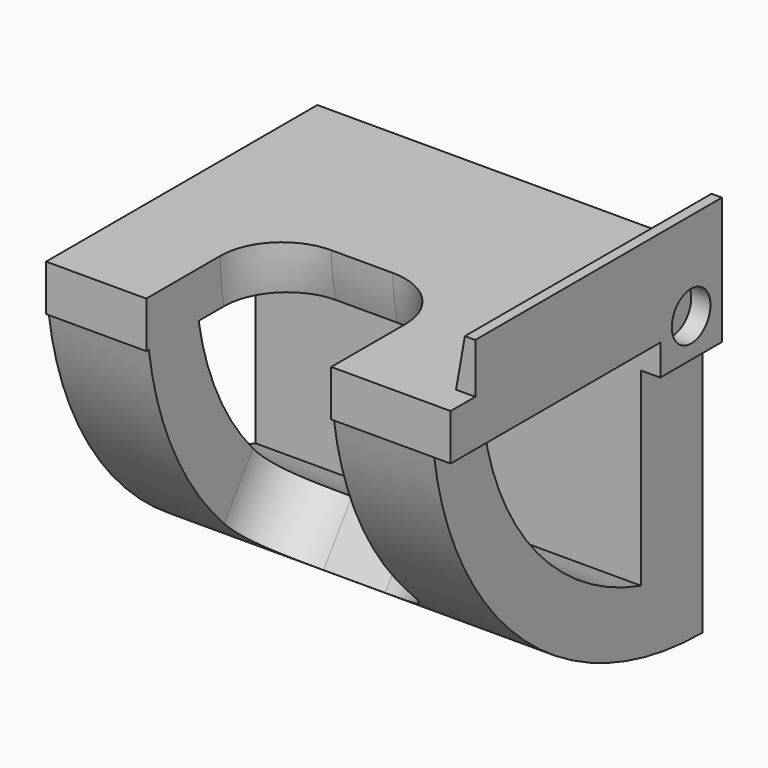
from build123d import *

# Parameters (mm, degrees)
F1_DEPTH      = 79.375
F4_DEPTH      = 19.05
F4_DEPTH_BACK = 19.05
F5_R          = 12.7
F7_W          = 9.525
F7_H          = 12.7
F8_DEPTH      = 3.175
F6_W          = 63.5
F6_H          = 10.3124
F6_R          = 4.9744809982
F9_DEPTH      = 3.9624
F10_SIZE2     = 1.818344
F10_SIZE      = 10.31239


# Not quite as in the source:
# - a fillet or chamfer is up to 0.001 mm smaller than in the source, because OpenCascade refuses the exact size


with BuildPart() as f1:
    # F0 (on Right) → F1 (new body)
    with BuildSketch(Plane.YZ):
        with BuildLine():
            Line((0, -9.525), (0, 0))
            Line((0, 0), (-57.15, 0))
            ThreePointArc((-57.15, 0), (-56.9498143774, -4.779240775), (-56.350659934, -9.525))
            Line((-56.350659934, -9.525), (-15.875, -9.525))
            Line((-15.875, -9.525), (0, -9.525))
        make_face()
        with BuildLine():
            ThreePointArc((-56.350659934, -9.525), (-56.9498143774, -4.779240775), (-57.15, 0))
            Line((-57.15, 0), (-69.85, 0))
            ThreePointArc((-69.85, 0), (-69.6866892703, -4.7736609169), (-69.1975207287, -9.525))
            Line((-69.1975207287, -9.525), (-56.350659934, -9.525))
        make_face()
        with BuildLine():
            Line((0, -57.15), (0, -9.525))
            Line((0, -9.525), (-15.875, -9.525))
            Line((-15.875, -9.525), (-15.875, -54.9008822789))
            ThreePointArc((-15.875, -54.9008822789), (-8.0167661111, -56.5849269781), (0, -57.15))
        make_face()
        with BuildLine():
            ThreePointArc((-69.1975207287, -9.525), (-69.6866892703, -4.7736609169), (-69.85, 0))
            Line((-69.85, 0), (-69.85, -9.525))
            Line((-69.85, -9.525), (-69.1975207287, -9.525))
        make_face()
        with BuildLine():
            ThreePointArc((-15.875, -54.9008822789), (-42.648319561, -38.042651572), (-56.350659934, -9.525))
            Line((-56.350659934, -9.525), (-69.1975207287, -9.525))
            ThreePointArc((-69.1975207287, -9.525), (-45.900442536, -52.6514185469), (0, -69.85))
            Line((0, -69.85), (0, -57.15))
            ThreePointArc((0, -57.15), (-8.0167661111, -56.5849269781), (-15.875, -54.9008822789))
        make_face()
    extrude(amount=-F1_DEPTH)

    # F3 (on offset) → F4 (cut, two sides)
    with BuildSketch(Plane.YZ.offset(-39.6875)) as f4_sk:
        with BuildLine():
            ThreePointArc((-21.853262225, -31.2096928874), (-33.7951127441, -17.5926221643), (-38.1, 0))
            Line((-38.1, 0), (-69.85, 0))
            Line((-69.85, 0), (-69.85, -9.525))
            Line((-69.85, -9.525), (-69.1975207287, -9.525))
            ThreePointArc((-69.1975207287, -9.525), (-59.6086170026, -36.4120210787), (-40.0643140791, -57.2177702936))
            Line((-40.0643140791, -57.2177702936), (-21.853262225, -31.2096928874))
        make_face()
        with BuildLine():
            ThreePointArc((-2.9503190018, -7.9502), (-3.1448391156, -6.5727258097), (-3.7131865837, -5.3029800181))
            Line((-3.7131865837, -5.3029800181), (-8.9719164583, -12.8132246066))
            ThreePointArc((-8.9719164583, -12.8132246066), (-4.7993720072, -11.8202337289), (-2.9503190018, -7.9502))
        make_face()
        with BuildLine():
            Line((-8.9719164583, -12.8132246066), (-3.7131865837, -5.3029800181))
            ThreePointArc((-3.7131865837, -5.3029800181), (-11.9996562789, -5.0969549164), (-8.9719164583, -12.8132246066))
        make_face()
    extrude(amount=-F4_DEPTH, mode=Mode.SUBTRACT)
    extrude(f4_sk.sketch, amount=F4_DEPTH_BACK, mode=Mode.SUBTRACT)

    # F5
    f5_edges = [f1.edges().sort_by_distance(p)[0] for p in [
        (-58.7375, -37.796331, -4.800764),
        (-58.7375, -36.422104, -52.016155),
        (-20.6375, -37.796331, -4.800764),
        (-20.6375, -36.422104, -52.016155),
    ]]
    fillet(f5_edges, radius=F5_R)

    # F7 (on face) → F8 (join)
    with BuildSketch(Plane(origin=(-79.375, 0, 0), x_dir=(0, -1, 0), z_dir=(-1, 0, 0))):
        with Locations((-4.7625, -63.5)):
            Rectangle(F7_W, F7_H)
    extrude(amount=-F8_DEPTH)

    # F6 (on face) → F9 (join)
    with BuildSketch(Plane.YZ):
        with Locations((-31.75, 5.1562)):
            Rectangle(F6_W, F6_H)
        Polygon((0, -15.875), (0, 0), (-63.5, 0), (-69.85, 0), (-69.85, -9.525), (-69.1975207287, -9.525), (-56.350659934, -9.525), (-15.875, -9.525), (-15.875, -15.875), align=None)
        with Locations((-7.9248, -7.9502)):
            Circle(F6_R, mode=Mode.SUBTRACT)
    extrude(amount=F9_DEPTH)

    # F10 (size 10.3124 and 1.8183543559 in the source; OpenCascade refuses exactly that, so slightly less here)
    f10_edges = [f1.edges().sort_by_distance(p)[0] for p in [
        (0, -31.75, 10.3124),
    ]]
    f10_side = f1.faces().sort_by_distance((0, -31.75, 5.1562))[0]
    chamfer(f10_edges, length=F10_SIZE, length2=F10_SIZE2, reference=f10_side)


solid = f1.part
